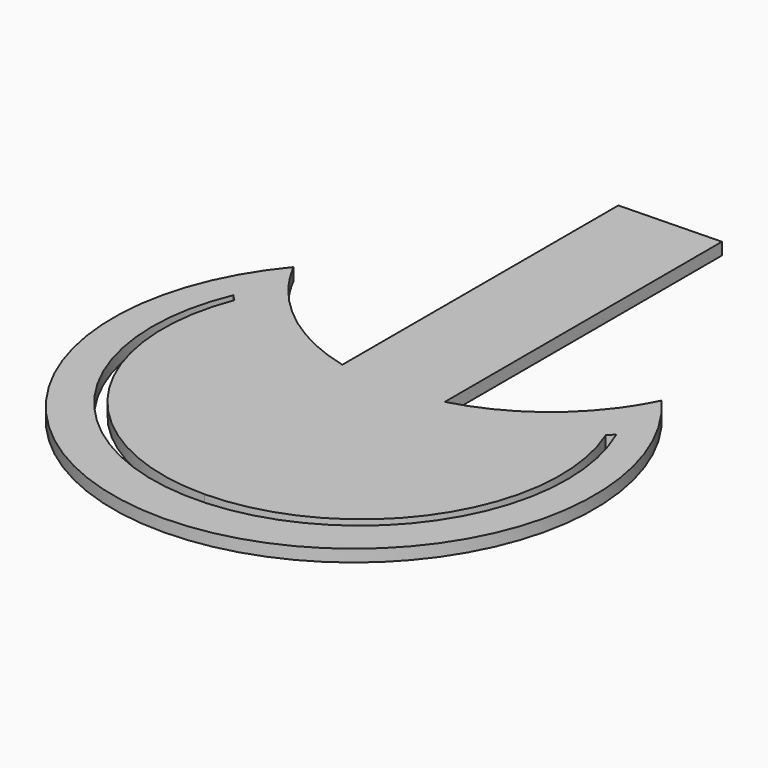
from build123d import *

# Parameters (mm, degrees)
F1_DEPTH = 6


# Not quite as in the source:
# - a feature names something its author has since deleted; it is built from what else it names


with BuildPart() as f1:
    # F0 (on Top) → F1 (new body)
    with BuildSketch(Plane.XY):
        with BuildLine():
            ThreePointArc((30.0553449159, -185.920695897), (17.5794063582, -188.4215241051), (4.8876879096, -189.3289751767))
            Line((4.8876879096, -189.3289751767), (5.7980329658, -303.75093242))
            ThreePointArc((5.7980329658, -303.75093242), (86.5273496986, -260.1965866309), (95.7430891745, -168.9317316034))
            ThreePointArc((95.7430891745, -168.9317316034), (90.8132652561, -158.6088748661), (84.7126559945, -148.9317316034))
            ThreePointArc((84.7126559945, -148.9317316034), (60.5005683745, -172.0314581931), (30.0553449159, -185.920695897))
        make_face()
        with BuildLine():
            ThreePointArc((98.5642250933, -165.9317316034), (90.8814208815, -262.6386931182), (5.8423814985, -309.3251329781))
            ThreePointArc((5.8423814985, -309.3251329781), (-79.8609699448, -263.9139469341), (-88.9966016407, -167.3542218927))
            ThreePointArc((-88.9966016407, -167.3542218927), (-83.929020631, -157.0369391236), (-77.7345321086, -147.3542218927))
            ThreePointArc((-77.7345321086, -147.3542218927), (-81.8805443881, -141.0981193513), (-85.5490516624, -134.5505784994))
            ThreePointArc((-85.5490516624, -134.5505784994), (6.1468085688, -329.3233337338), (94.4628409087, -132.9949471034))
            ThreePointArc((94.4628409087, -132.9949471034), (90.9080384927, -139.6049105385), (86.8707656456, -145.9317316034))
            ThreePointArc((86.8707656456, -145.9317316034), (93.2862540801, -155.5991937575), (98.5642250933, -165.9317316034))
        make_face()
        with BuildLine():
            Line((5.7980329658, -303.75093242), (4.8876879096, -189.3289751767))
            ThreePointArc((4.8876879096, -189.3289751767), (-7.6794152519, -188.6448310467), (-20.0630018523, -186.3982963877))
            Line((-20.0630018523, -186.3982963877), (-20.0630018523, -187.4059048465))
            Line((-20.0630018523, -187.4059048465), (-20.1645397489, -186.3731772774))
            ThreePointArc((-20.1645397489, -186.3731772774), (-50.8661384709, -173.027578246), (-75.4956347969, -150.3542218927))
            ThreePointArc((-75.4956347969, -150.3542218927), (-81.3750972509, -160.0468085115), (-86.0943708707, -170.3542218927))
            ThreePointArc((-86.0943708707, -170.3542218927), (-75.4947572543, -261.4016255971), (5.7980329658, -303.75093242))
        make_face()
        with BuildLine():
            Line((-88.9966016407, -167.3542218927), (-86.0943708707, -170.3542218927))
            ThreePointArc((-86.0943708707, -170.3542218927), (-81.3750972509, -160.0468085115), (-75.4956347969, -150.3542218927))
            ThreePointArc((-75.4956347969, -150.3542218927), (-76.6290258855, -148.8646271178), (-77.7345321086, -147.3542218927))
            ThreePointArc((-77.7345321086, -147.3542218927), (-83.929020631, -157.0369391236), (-88.9966016407, -167.3542218927))
        make_face()
        with BuildLine():
            ThreePointArc((84.7126559945, -148.9317316034), (90.8132652561, -158.6088748661), (95.7430891745, -168.9317316034))
            Line((95.7430891745, -168.9317316034), (98.5642250933, -165.9317316034))
            ThreePointArc((98.5642250933, -165.9317316034), (93.2862540801, -155.5991937575), (86.8707656456, -145.9317316034))
            ThreePointArc((86.8707656456, -145.9317316034), (85.8054753664, -147.4416334036), (84.7126559945, -148.9317316034))
        make_face()
        with BuildLine():
            ThreePointArc((-20.0630018523, -186.3982963877), (-7.6794152519, -188.6448310467), (4.8876879096, -189.3289751767))
            ThreePointArc((4.8876879096, -189.3289751767), (17.5794063582, -188.4215241051), (30.0553449159, -185.920695897))
            Line((30.0553449159, -185.920695897), (29.9369981477, -15.103455868))
            Line((29.9369981477, -15.103455868), (-20.0630018523, -16.3942482322))
            Line((-20.0630018523, -16.3942482322), (-20.0630018523, -186.3982963877))
        make_face()
    extrude(amount=F1_DEPTH)


solid = f1.part
